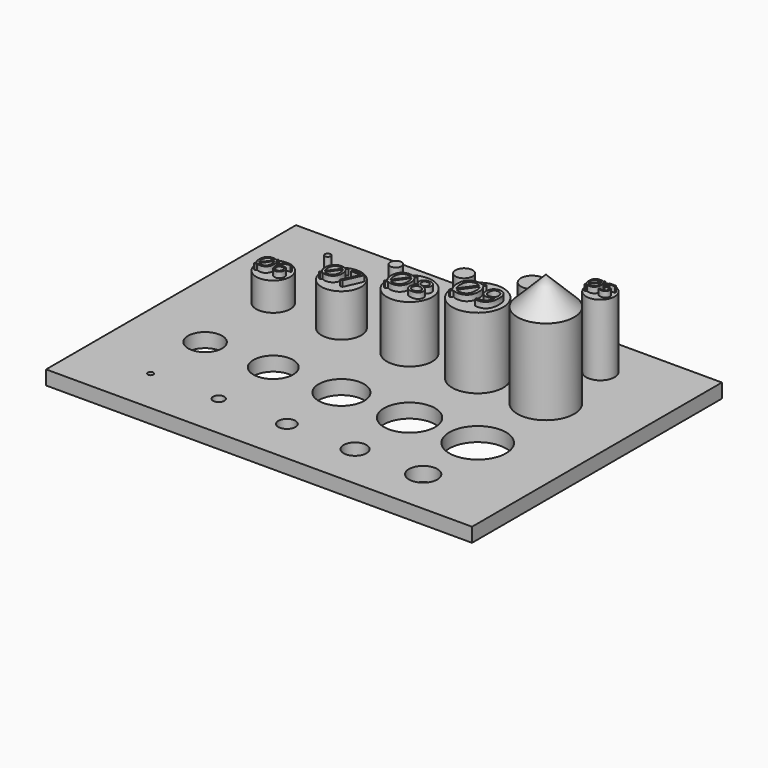
from build123d import *

# Parameters (mm, degrees)
F0_W          = 75
F0_H          = 55
F0_R          = 0.5
F0_R_2        = 1
F0_R_3        = 1.5
F0_R_4        = 3
F0_R_5        = 3.5
F0_R_6        = 4
F0_R_7        = 2
F0_R_8        = 2.5
F0_R_9        = 4.5
F0_R_10       = 5
F1_DEPTH      = 2.5
F2_DEPTH      = 5
F3_DEPTH      = 7.5
F4_DEPTH      = 10
F5_DEPTH      = 12.5
F6_DEPTH      = 15
F7_DEPTH      = 7.5
F8_DEPTH      = 10
F9_DEPTH      = 12.5
F10_DEPTH     = 15
F11_DEPTH     = 22.5
F12_SIZE      = 5
F13_TEXT_SIZE = 5.8428281361
F14_DEPTH     = 1
F15_TEXT_SIZE = 5.1880413548
F16_DEPTH     = 1
F17_TEXT_SIZE = 4.5370967253
F18_DEPTH     = 1
F19_TEXT_SIZE = 3.8844162551
F20_DEPTH     = 1
F21_TEXT_SIZE = 3.2533068016
F22_DEPTH     = 1


# Not quite as in the source:
# - Text() gives the source's letters only with a copy of the font that has no kerning and outlines rounded to 1/6400 em; it was checked with that copy


with BuildPart() as f1:
    # F0 (on Top) → F1 (new body)
    with BuildSketch(Plane.XY):
        Rectangle(F0_W, F0_H)
        with Locations((-25.5, -19.5)):
            Circle(F0_R, mode=Mode.SUBTRACT)
        with Locations((-13.5, -19.5)):
            Circle(F0_R_2, mode=Mode.SUBTRACT)
        with Locations((-1.5, -19.5)):
            Circle(F0_R_3, mode=Mode.SUBTRACT)
        with Locations((-25.5, -7.5)):
            Circle(F0_R_4, mode=Mode.SUBTRACT)
        with Locations((-13.5, -7.5)):
            Circle(F0_R_5, mode=Mode.SUBTRACT)
        with Locations((-1.5, -7.5)):
            Circle(F0_R_6, mode=Mode.SUBTRACT)
        with Locations((10.5, -19.5)):
            Circle(F0_R_7, mode=Mode.SUBTRACT)
        with Locations((22.5, -19.5)):
            Circle(F0_R_8, mode=Mode.SUBTRACT)
        with Locations((10.5, -7.5)):
            Circle(F0_R_9, mode=Mode.SUBTRACT)
        with Locations((22.5, -7.5)):
            Circle(F0_R_10, mode=Mode.SUBTRACT)
        with Locations((-25.5, 7.5)):
            Circle(F0_R_4, mode=Mode.SUBTRACT)
        with Locations((-13.5, 7.5)):
            Circle(F0_R_5, mode=Mode.SUBTRACT)
        with Locations((-1.5, 7.5)):
            Circle(F0_R_6, mode=Mode.SUBTRACT)
        with Locations((-25.5, 19.5)):
            Circle(F0_R, mode=Mode.SUBTRACT)
        with Locations((-13.5, 19.5)):
            Circle(F0_R_2, mode=Mode.SUBTRACT)
        with Locations((-1.5, 19.5)):
            Circle(F0_R_3, mode=Mode.SUBTRACT)
        with Locations((10.5, 7.5)):
            Circle(F0_R_9, mode=Mode.SUBTRACT)
        with Locations((22.5, 7.5)):
            Circle(F0_R_10, mode=Mode.SUBTRACT)
        with Locations((10.5, 19.5)):
            Circle(F0_R_7, mode=Mode.SUBTRACT)
        with Locations((22.5, 19.5)):
            Circle(F0_R_8, mode=Mode.SUBTRACT)
    extrude(amount=F1_DEPTH)

    # F0 (on Top) → F2 (join)
    with BuildSketch(Plane.XY):
        with Locations((-25.5, 19.5)):
            Circle(F0_R)
    extrude(amount=F2_DEPTH)

    # F0 (on Top) → F3 (join)
    with BuildSketch(Plane.XY):
        with Locations((-13.5, 19.5)):
            Circle(F0_R_2)
    extrude(amount=F3_DEPTH)

    # F0 (on Top) → F4 (join)
    with BuildSketch(Plane.XY):
        with Locations((-1.5, 19.5)):
            Circle(F0_R_3)
    extrude(amount=F4_DEPTH)

    # F0 (on Top) → F5 (join)
    with BuildSketch(Plane.XY):
        with Locations((10.5, 19.5)):
            Circle(F0_R_7)
    extrude(amount=F5_DEPTH)

    # F0 (on Top) → F6 (join)
    with BuildSketch(Plane.XY):
        with Locations((22.5, 19.5)):
            Circle(F0_R_8)
    extrude(amount=F6_DEPTH)

    # F0 (on Top) → F7 (join)
    with BuildSketch(Plane.XY):
        with Locations((-25.5, 7.5)):
            Circle(F0_R_4)
    extrude(amount=F7_DEPTH)

    # F0 (on Top) → F8 (join)
    with BuildSketch(Plane.XY):
        with Locations((-13.5, 7.5)):
            Circle(F0_R_5)
    extrude(amount=F8_DEPTH)

    # F0 (on Top) → F9 (join)
    with BuildSketch(Plane.XY):
        with Locations((-1.5, 7.5)):
            Circle(F0_R_6)
    extrude(amount=F9_DEPTH)

    # F0 (on Top) → F10 (join)
    with BuildSketch(Plane.XY):
        with Locations((10.5, 7.5)):
            Circle(F0_R_9)
    extrude(amount=F10_DEPTH)

    # F0 (on Top) → F11 (join)
    with BuildSketch(Plane.XY):
        with Locations((22.5, 7.5)):
            Circle(F0_R_10)
    extrude(amount=F11_DEPTH)

    # F12
    f12_edges = [f1.edges().sort_by_distance(p)[0] for p in [
        (17.5, 7.5, 22.5),
    ]]
    chamfer(f12_edges, length=F12_SIZE)

    # F13 (on face) → F14 (join)
    with BuildSketch(Plane.XY.offset(15)):
        with Locations((6.521855687, 5.396581871)):
            Text('Ø9', F13_TEXT_SIZE, font='Open Sans', text_align=(TextAlign.LEFT, TextAlign.BOTTOM))
    extrude(amount=F14_DEPTH)

    # F15 (on face) → F16 (join)
    with BuildSketch(Plane.XY.offset(12.5)):
        with Locations((-5.0371903831, 5.6323051123)):
            Text('Ø8', F15_TEXT_SIZE, font='Open Sans', text_align=(TextAlign.LEFT, TextAlign.BOTTOM))
    extrude(amount=F16_DEPTH)

    # F17 (on face) → F18 (join)
    with BuildSketch(Plane.XY.offset(10)):
        with Locations((-16.595505133, 5.8666451789)):
            Text('Ø7', F17_TEXT_SIZE, font='Open Sans', text_align=(TextAlign.LEFT, TextAlign.BOTTOM))
    extrude(amount=F18_DEPTH)

    # F19 (on face) → F20 (join)
    with BuildSketch(Plane.XY.offset(7.5)):
        with Locations((-28.1541487943, 6.1016101482)):
            Text('Ø6', F19_TEXT_SIZE, font='Open Sans', text_align=(TextAlign.LEFT, TextAlign.BOTTOM))
    extrude(amount=F20_DEPTH)

    # F21 (on face) → F22 (join)
    with BuildSketch(Plane.XY.offset(15)):
        with Locations((20.2913096792, 18.3288095514)):
            Text('Ø5', F21_TEXT_SIZE, font='Open Sans', text_align=(TextAlign.LEFT, TextAlign.BOTTOM))
    extrude(amount=F22_DEPTH)


solid = f1.part
